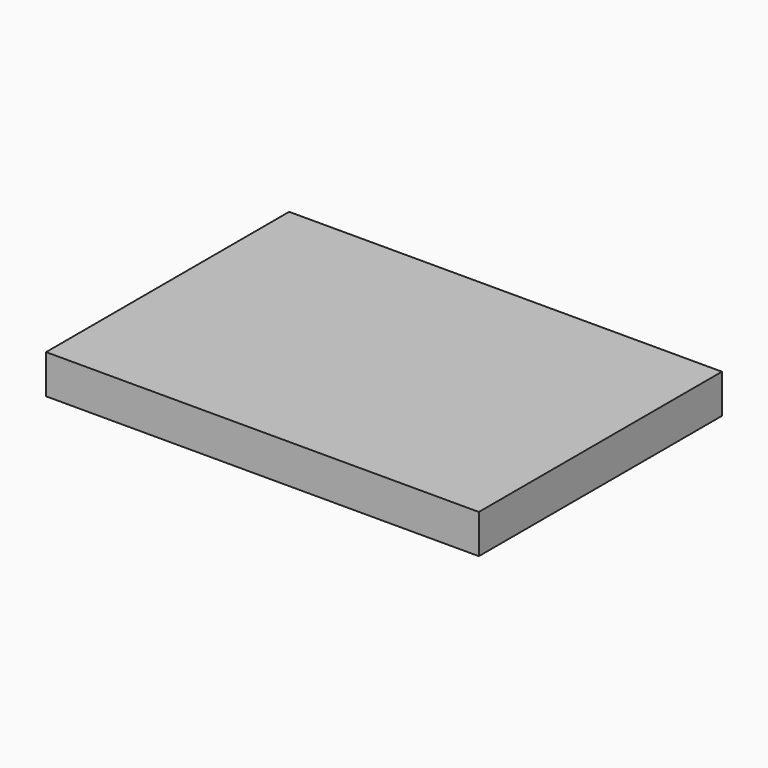
from build123d import *

# Parameters (mm, degrees)
F0_W     = 500
F0_H     = 350.9934146229
F1_DEPTH = 22.5


# Not quite as in the source:
# - a feature of the source that left no trace in its solid (it failed there, or was rolled back) is left out
# - the program builds the solid bodies; features that only make, move or delete a surface that nothing else refers to are left out


with BuildPart() as f1:
    # F0 (on Top) → F1 (new body, symmetric)
    with BuildSketch(Plane.XY):
        Rectangle(F0_W, F0_H)
    extrude(amount=F1_DEPTH, both=True)


solid = f1.part
